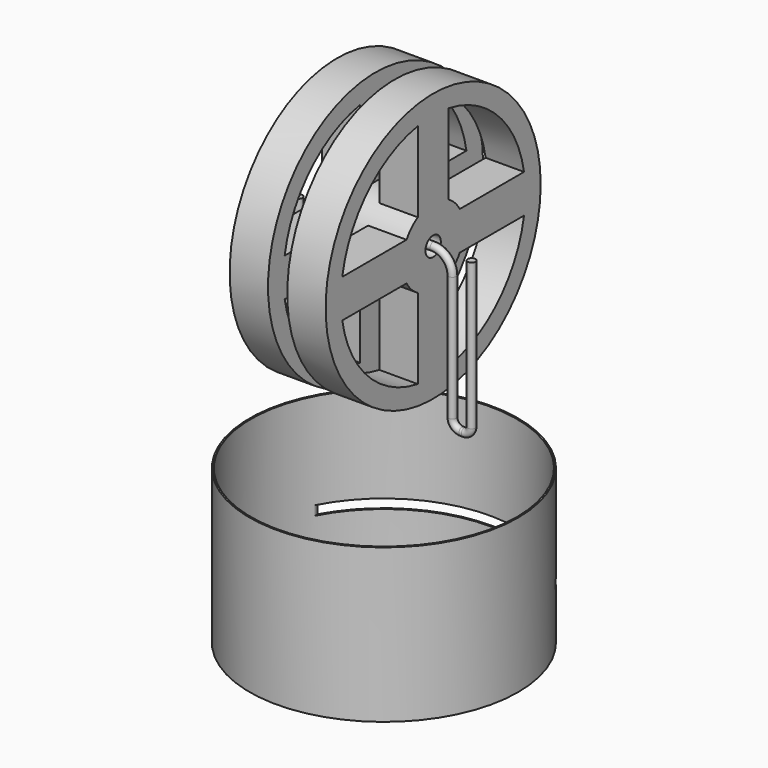
from build123d import *

# Parameters (mm, degrees)
F0_R      = 44.45
F0_R_2    = 3.175
F1_DEPTH  = 12.7
F2_R      = 3.175
F3_DEPTH  = 6.35
F4_R      = 44.45
F4_R_2    = 3.175
F5_DEPTH  = 12.7
F6_R      = 1.016
F7_DEPTH  = 25.4
F8_R      = 10.2329396238
F8_R_2    = 1.016
F9_DEPTH  = 55.88
F12_R     = 1.27
F15_R     = 44.45
F15_R_2   = 43.942
F16_DEPTH = 50.8
F18_W     = 76.2
F18_H     = 3.0743540772
F19_DEPTH = 50.8


with BuildPart() as f1:
    # F0 (on Right) → F1 (new body)
    with BuildSketch(Plane.YZ):
        Circle(F0_R)
        with BuildLine():
            ThreePointArc((37.5707122885, 6.3286316164), (37.9674474925, 3.1753631138), (38.1, 0))
            ThreePointArc((38.1, 0), (37.9656351859, -3.1969587), (37.5634884552, -6.3713683836))
            ThreePointArc((37.5634884552, -6.3713683836), (26.9331048739, -26.9484296732), (6.35, -37.5671066227))
            ThreePointArc((6.35, -37.5671066227), (0, -38.1), (-6.35, -37.5671066227))
            ThreePointArc((-6.35, -37.5671066227), (-26.9331048739, -26.9484296732), (-37.5634884552, -6.3713683836))
            ThreePointArc((-37.5634884552, -6.3713683836), (-38.0999938366, -0.0216714965), (-37.5707122885, 6.3286316164))
            ThreePointArc((-37.5707122885, 6.3286316164), (-26.9484289368, 26.9331056107), (-6.35, 37.5671066227))
            ThreePointArc((-6.35, 37.5671066227), (0, 38.1), (6.35, 37.5671066227))
            ThreePointArc((6.35, 37.5671066227), (26.9484289368, 26.9331056107), (37.5707122885, 6.3286316164))
        make_face(mode=Mode.SUBTRACT)
        with BuildLine():
            Line((6.35, 10.9985226281), (6.35, 37.5671066227))
            ThreePointArc((6.35, 37.5671066227), (0, 38.1), (-6.35, 37.5671066227))
            Line((-6.35, 37.5671066227), (-6.35, 10.9985226281))
            ThreePointArc((-6.35, 10.9985226281), (0, 12.7), (6.35, 10.9985226281))
        make_face()
        with BuildLine():
            Line((-11.0108320241, 6.3286316164), (-37.5707122885, 6.3286316164))
            ThreePointArc((-37.5707122885, 6.3286316164), (-38.0999938366, -0.0216714965), (-37.5634884552, -6.3713683836))
            Line((-37.5634884552, -6.3713683836), (-10.986157878, -6.3713683836))
            ThreePointArc((-10.986157878, -6.3713683836), (-12.699976031, -0.0246740995), (-11.0108320241, 6.3286316164))
        make_face()
        with BuildLine():
            ThreePointArc((37.5634884552, -6.3713683836), (37.9656351859, -3.1969587), (38.1, 0))
            ThreePointArc((38.1, 0), (37.9674474925, 3.1753631138), (37.5707122885, 6.3286316164))
            Line((37.5707122885, 6.3286316164), (11.0108320241, 6.3286316164))
            ThreePointArc((11.0108320241, 6.3286316164), (12.2704434864, 3.2750903265), (12.7, 0))
            ThreePointArc((12.7, 0), (12.2640573435, -3.2989236843), (10.986157878, -6.3713683836))
            Line((10.986157878, -6.3713683836), (37.5634884552, -6.3713683836))
        make_face()
        with BuildLine():
            ThreePointArc((-6.35, -37.5671066227), (0, -38.1), (6.35, -37.5671066227))
            Line((6.35, -37.5671066227), (6.35, -11.9964098558))
            Line((6.35, -11.9964098558), (6.35, -10.9985226281))
            ThreePointArc((6.35, -10.9985226281), (0, -12.7), (-6.35, -10.9985226281))
            Line((-6.35, -10.9985226281), (-6.35, -37.5671066227))
        make_face()
        with BuildLine():
            ThreePointArc((12.7, 0), (12.2704434864, 3.2750903265), (11.0108320241, 6.3286316164))
            ThreePointArc((11.0108320241, 6.3286316164), (8.9889706117, 8.9715331656), (6.35, 10.9985226281))
            ThreePointArc((6.35, 10.9985226281), (0, 12.7), (-6.35, 10.9985226281))
            ThreePointArc((-6.35, 10.9985226281), (-8.9889706117, 8.9715331656), (-11.0108320241, 6.3286316164))
            ThreePointArc((-11.0108320241, 6.3286316164), (-12.699976031, -0.0246740995), (-10.986157878, -6.3713683836))
            ThreePointArc((-10.986157878, -6.3713683836), (-8.9715233708, -8.9889803875), (-6.35, -10.9985226281))
            ThreePointArc((-6.35, -10.9985226281), (0, -12.7), (6.35, -10.9985226281))
            ThreePointArc((6.35, -10.9985226281), (8.9715233708, -8.9889803875), (10.986157878, -6.3713683836))
            ThreePointArc((10.986157878, -6.3713683836), (12.2640573435, -3.2989236843), (12.7, 0))
        make_face()
        Circle(F0_R_2, mode=Mode.SUBTRACT)
    extrude(amount=F1_DEPTH)

    # F2 (on face) → F3 (join)
    with BuildSketch(Plane.YZ.offset(12.7)):
        with BuildLine():
            ThreePointArc((10.986157878, -6.3713683836), (12.2640573435, -3.2989236843), (12.7, 0))
            ThreePointArc((12.7, 0), (12.2704434864, 3.2750903265), (11.0108320241, 6.3286316164))
            ThreePointArc((11.0108320241, 6.3286316164), (8.9889706117, 8.9715331656), (6.35, 10.9985226281))
            ThreePointArc((6.35, 10.9985226281), (0, 12.7), (-6.35, 10.9985226281))
            ThreePointArc((-6.35, 10.9985226281), (-8.9889706117, 8.9715331656), (-11.0108320241, 6.3286316164))
            ThreePointArc((-11.0108320241, 6.3286316164), (-12.699976031, -0.0246740995), (-10.986157878, -6.3713683836))
            ThreePointArc((-10.986157878, -6.3713683836), (-8.9715233708, -8.9889803875), (-6.35, -10.9985226281))
            ThreePointArc((-6.35, -10.9985226281), (0, -12.7), (6.35, -10.9985226281))
            ThreePointArc((6.35, -10.9985226281), (8.9715233708, -8.9889803875), (10.986157878, -6.3713683836))
        make_face()
        Circle(F2_R, mode=Mode.SUBTRACT)
    extrude(amount=F3_DEPTH)

    # F4 (on face) → F5 (join)
    with BuildSketch(Plane.YZ.offset(19.05)):
        Circle(F4_R)
        with BuildLine():
            ThreePointArc((37.5671066227, 6.35), (37.9665429182, 3.1861605167), (38.1, 0))
            ThreePointArc((38.1, 0), (37.9665429182, -3.1861605167), (37.5671066227, -6.35))
            ThreePointArc((37.5671066227, -6.35), (26.9407683632, -26.9407683632), (6.35, -37.5671066227))
            ThreePointArc((6.35, -37.5671066227), (0, -38.1), (-6.35, -37.5671066227))
            ThreePointArc((-6.35, -37.5671066227), (-26.9407683632, -26.9407683632), (-37.5671066227, -6.35))
            ThreePointArc((-37.5671066227, -6.35), (-38.1, 0), (-37.5671066227, 6.35))
            ThreePointArc((-37.5671066227, 6.35), (-26.9407683632, 26.9407683632), (-6.35, 37.5671066227))
            ThreePointArc((-6.35, 37.5671066227), (0, 38.1), (6.35, 37.5671066227))
            ThreePointArc((6.35, 37.5671066227), (26.9407683632, 26.9407683632), (37.5671066227, 6.35))
        make_face(mode=Mode.SUBTRACT)
        with BuildLine():
            ThreePointArc((10.9985226281, 6.35), (8.9802561211, 8.9802561211), (6.35, 10.9985226281))
            ThreePointArc((6.35, 10.9985226281), (0, 12.7), (-6.35, 10.9985226281))
            ThreePointArc((-6.35, 10.9985226281), (-8.9802561211, 8.9802561211), (-10.9985226281, 6.35))
            ThreePointArc((-10.9985226281, 6.35), (-12.7, 0), (-10.9985226281, -6.35))
            ThreePointArc((-10.9985226281, -6.35), (-8.9802561211, -8.9802561211), (-6.35, -10.9985226281))
            ThreePointArc((-6.35, -10.9985226281), (0, -12.7), (6.35, -10.9985226281))
            ThreePointArc((6.35, -10.9985226281), (8.9802561211, -8.9802561211), (10.9985226281, -6.35))
            ThreePointArc((10.9985226281, -6.35), (12.2672579939, -3.2870018728), (12.7, 0))
            ThreePointArc((12.7, 0), (12.2672579939, 3.2870018728), (10.9985226281, 6.35))
        make_face()
        Circle(F4_R_2, mode=Mode.SUBTRACT)
        with BuildLine():
            Line((6.35, 10.9985226281), (6.35, 37.5671066227))
            ThreePointArc((6.35, 37.5671066227), (0, 38.1), (-6.35, 37.5671066227))
            Line((-6.35, 37.5671066227), (-6.35, 10.9985226281))
            ThreePointArc((-6.35, 10.9985226281), (0, 12.7), (6.35, 10.9985226281))
        make_face()
        with BuildLine():
            ThreePointArc((37.5671066227, -6.35), (37.9665429182, -3.1861605167), (38.1, 0))
            ThreePointArc((38.1, 0), (37.9665429182, 3.1861605167), (37.5671066227, 6.35))
            Line((37.5671066227, 6.35), (21.1177552809, 6.35))
            Line((21.1177552809, 6.35), (10.9985226281, 6.35))
            ThreePointArc((10.9985226281, 6.35), (12.2672579939, 3.2870018728), (12.7, 0))
            ThreePointArc((12.7, 0), (12.2672579939, -3.2870018728), (10.9985226281, -6.35))
            Line((10.9985226281, -6.35), (21.1177552809, -6.35))
            Line((21.1177552809, -6.35), (37.5671066227, -6.35))
        make_face()
        with BuildLine():
            ThreePointArc((-6.35, -37.5671066227), (0, -38.1), (6.35, -37.5671066227))
            Line((6.35, -37.5671066227), (6.35, -10.9985226281))
            ThreePointArc((6.35, -10.9985226281), (0, -12.7), (-6.35, -10.9985226281))
            Line((-6.35, -10.9985226281), (-6.35, -37.5671066227))
        make_face()
        with BuildLine():
            Line((-10.9985226281, 6.35), (-37.5671066227, 6.35))
            ThreePointArc((-37.5671066227, 6.35), (-38.1, 0), (-37.5671066227, -6.35))
            Line((-37.5671066227, -6.35), (-10.9985226281, -6.35))
            ThreePointArc((-10.9985226281, -6.35), (-12.7, 0), (-10.9985226281, 6.35))
        make_face()
    extrude(amount=F5_DEPTH)


with BuildPart() as f7:
    # F6 (on face) → F7 (new body)
    with BuildSketch(Plane.YZ.offset(31.75)):
        Circle(F6_R)
    extrude(amount=F7_DEPTH)

    # F8 (on face) → F9 (join)
    with BuildSketch(Plane(origin=(31.75, 0, 0), x_dir=(0, -1, 0), z_dir=(-1, 0, 0))):
        Circle(F8_R)
        Circle(F8_R_2, mode=Mode.SUBTRACT)
    extrude(amount=F9_DEPTH)


with BuildPart() as f13:
    # F13: sweep along a path in F11
    with BuildLine(Plane.XZ) as f13_path:
        Line((-12.7, 0), (-12.7, -48.4160261258))
        ThreePointArc((-12.7, -48.4160261258), (-12.0017502184, -50.1017502184), (-10.3160261258, -50.8))
        Line((-10.3160261258, -50.8), (-9.525, -50.8))
        ThreePointArc((-9.525, -50.8), (-7.2799359697, -49.8700640303), (-6.35, -47.625))
        Line((-6.35, -47.625), (-6.35, -6.35))
        ThreePointArc((-6.35, -6.35), (-4.4901280605, -1.8598719395), (0, 0))
        Line((0, 0), (31.75, 0))
        ThreePointArc((31.75, 0), (36.2401280605, -1.8598719395), (38.1, -6.35))
        Line((38.1, -6.35), (38.1, -47.625))
        ThreePointArc((38.1, -47.625), (39.0299359697, -49.8700640303), (41.275, -50.8))
        Line((41.275, -50.8), (42.0660261258, -50.8))
        ThreePointArc((42.0660261258, -50.8), (43.7517502184, -50.1017502184), (44.45, -48.4160261258))
        Line((44.45, -48.4160261258), (44.45, 0))
    # F12 (on Top) → F13 (sweep)
    with BuildSketch(Plane.XY):
        with Locations((-12.7, 0)):
            Circle(F12_R)
    sweep(path=f13_path.line)


with BuildPart() as f16:
    # F15 (on offset) → F16 (new body)
    with BuildSketch(Plane(origin=(0, 0, -69.8713683836), x_dir=(1, 0, 0), z_dir=(0, 0, -1))):
        with Locations((15.4646732695, 0)):
            Circle(F15_R)
        with Locations((15.4646732695, 0)):
            Circle(F15_R_2, mode=Mode.SUBTRACT)
    extrude(amount=F16_DEPTH)

    # F18 (on offset) → F19 (cut)
    with BuildSketch(Plane.XZ.offset(-63.5)):
        with Locations((14.5520862598, -103.1585454222)):
            Rectangle(F18_W, F18_H)
    extrude(amount=F19_DEPTH, mode=Mode.SUBTRACT)


solid = Compound([f1.part, f13.part, f16.part])
